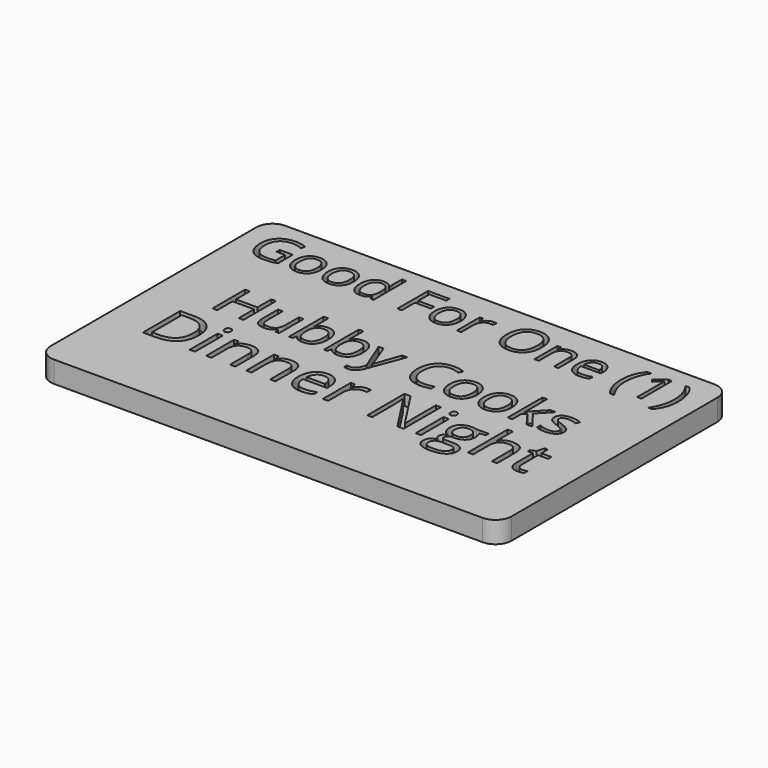
from build123d import *

# Parameters (mm, degrees)
F1_DEPTH       = 4
F2_TEXT_SIZE   = 10.0013673744
F3_DEPTH       = 2
F4_TEXT_SIZE   = 10.6595783623
F4_TEXT_SIZE_2 = 12.1665716873
F5_DEPTH       = 2


# Not quite as in the source:
# - Text() gives the source's letters only with a copy of the font that has no kerning and outlines rounded to 1/6400 em; it was checked with that copy


with BuildPart() as f1:
    # F0 (on Top) → F1 (new body)
    with BuildSketch(Plane.XY):
        with BuildLine():
            ThreePointArc((43, 24), (42.1213203436, 26.1213203436), (40, 27))
            Line((40, 27), (-40, 27))
            ThreePointArc((-40, 27), (-42.1213203436, 26.1213203436), (-43, 24))
            Line((-43, 24), (-43, -24))
            ThreePointArc((-43, -24), (-42.1213203436, -26.1213203436), (-40, -27))
            Line((-40, -27), (40, -27))
            ThreePointArc((40, -27), (42.1213203436, -26.1213203436), (43, -24))
            Line((43, -24), (43, 24))
        make_face()
    extrude(amount=F1_DEPTH)

    # F2 (on face) → F3 (cut)
    with BuildSketch(Plane.XY.offset(4)):
        with Locations((-40, 16.7990154904)):
            Text('Good For One (1)', F2_TEXT_SIZE, font='Open Sans', text_align=(TextAlign.LEFT, TextAlign.BOTTOM))
    extrude(amount=-F3_DEPTH, mode=Mode.SUBTRACT)

    # F4 (on face) → F5 (cut)
    with BuildSketch(Plane.XY.offset(4)):
        with Locations((-33.048856821, 0)):
            Text('Hubby Cooks', F4_TEXT_SIZE, font='Open Sans', text_align=(TextAlign.LEFT, TextAlign.BOTTOM))
        with Locations((-36.370501118, -12.2400680557)):
            Text('Dinner Night', F4_TEXT_SIZE_2, font='Open Sans', text_align=(TextAlign.LEFT, TextAlign.BOTTOM))
    extrude(amount=-F5_DEPTH, mode=Mode.SUBTRACT)


solid = f1.part
